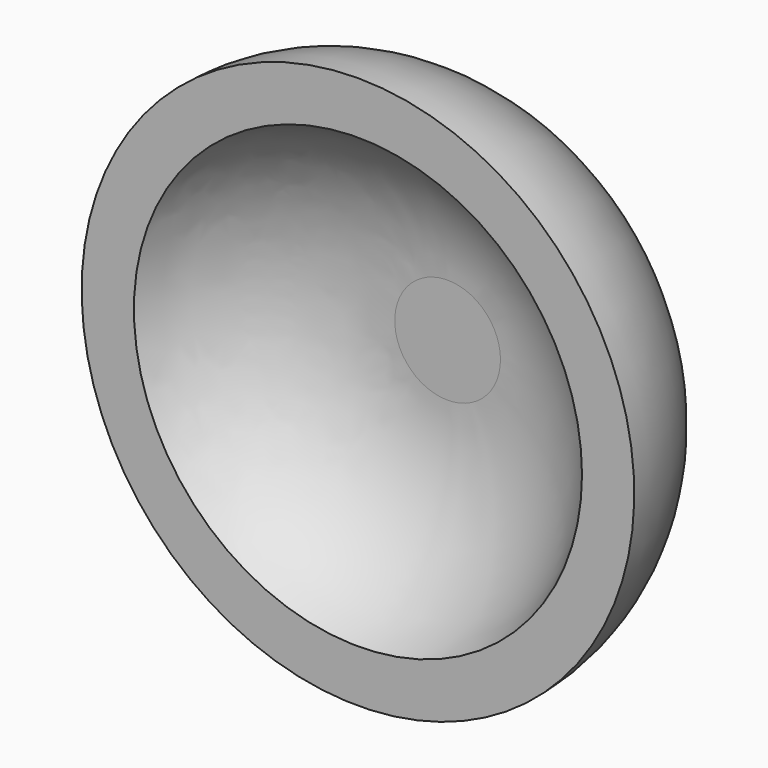
from build123d import *

# Parameters (mm, degrees)
F1_DEPTH = 25.4
F2_R     = 25.39999
F3_R     = 30.4669012051
F4_DEPTH = 15.24


# Not quite as in the source:
# - a fillet or chamfer that OpenCascade refuses, or shapes differently, is made with other operations: its cross-section is extruded or revolved along the edge and cut away or added
# - a fillet or chamfer is up to 0.001 mm smaller than in the source, because OpenCascade refuses the exact size


with BuildPart() as f1:
    # F0 (on Front) → F1 (new body)
    with BuildSketch(Plane.XZ):
        with BuildLine():
            ThreePointArc((20.0883221204, -31.7517811512), (32.9126956238, -18.1237622657), (37.5728132017, 0))
            ThreePointArc((37.5728132017, 0), (-18.1237622657, 32.9126956238), (-20.0883221204, -31.7517811512))
            ThreePointArc((-20.0883221204, -31.7517811512), (0, -37.5728132017), (20.0883221204, -31.7517811512))
        make_face()
    extrude(amount=F1_DEPTH)

    # F2 (radius 25.4 in the source; OpenCascade refuses exactly that, so slightly less here)
    f2_edges = [f1.edges().sort_by_distance(p)[0] for p in [
        (20.088322, 0, 31.751781),
    ]]
    fillet(f2_edges, radius=F2_R)

    # F3 (on face) → F4 (cut)
    with BuildSketch(Plane.XZ.offset(25.4)):
        Circle(F3_R)
    extrude(amount=-F4_DEPTH, mode=Mode.SUBTRACT)

    # F5: fillet of radius 25.4 on 1 edges, made by hand

    # F5_s1 → F5_t2 (revolve)
    with BuildSketch(Plane.XY):
        with BuildLine():
            ThreePointArc((30.4669012051, -25.4), (21.0995696353, -14.308835326), (7.1874166747, -10.16))
            Line((7.1874166747, -10.16), (30.4669012051, -10.16))
            Line((30.4669012051, -10.16), (30.4669012051, -25.4))
        make_face()
    revolve(axis=Axis((0, -10.16, 0), (0, -1, 0)))


solid = f1.part
